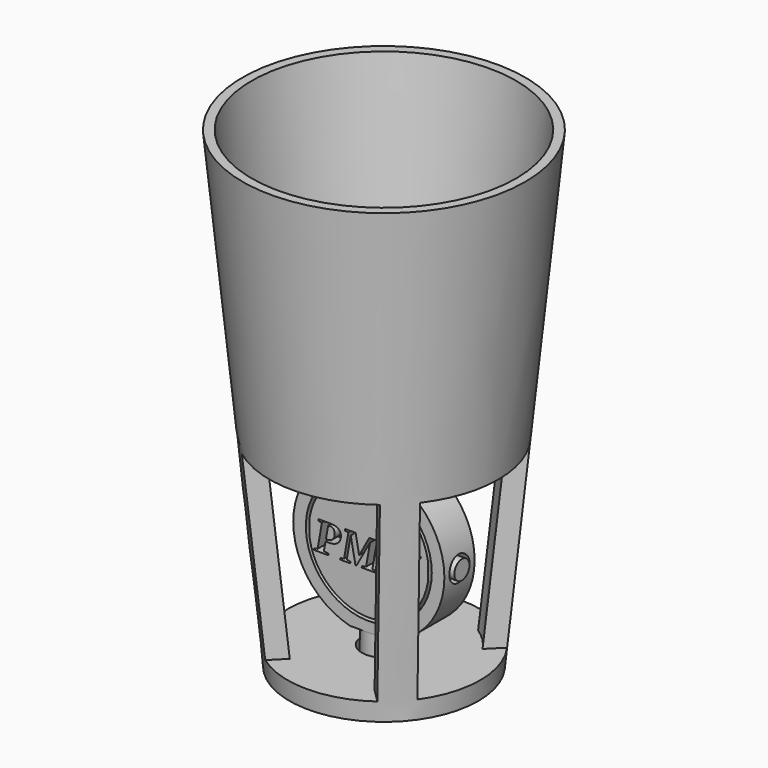
from build123d import *

# Parameters (mm, degrees)
F3_DEPTH      = 29
F4_R          = 3.5
F5_DEPTH      = 2
F5_DEPTH_BACK = 31
F6_R          = 10
F7_DEPTH      = 3
F8_R          = 2
F9_DEPTH      = 15
F11_DEPTH     = 3
F16_TEXT_SIZE = 6.9444444444
F17_DEPTH     = 2
F18_TEXT_SIZE = 6.9444444444
F19_DEPTH     = 2


# Not quite as in the source:
# - Text() gives the source's letters only with a copy of the font that has no kerning and outlines rounded to 1/6400 em; it was checked with that copy


with BuildPart() as f1:
    # F0 (on Front) → F1 (revolve)
    with BuildSketch(Plane.XZ):
        Polygon((0, 3), (0, 0), (15, 0), (22.447081343, 75), (21, 75), (17.0282232837, 35), (0, 35), (0, 32), (15.1626685751, 32), (12.2831304558, 3), align=None)
    revolve(axis=Axis((0, 0, 33.5), (0, 0, 1)))

    # F2 (on face) → F3 (cut)
    with BuildSketch(Plane.XY.offset(3)):
        with BuildLine():
            Line((12.2634482474, 15.7989821534), (15.6845353346, 19.2200692405))
            ThreePointArc((15.6845353346, 19.2200692405), (0, 24.8075736474), (-15.6845353346, 19.2200692405))
            Line((-15.6845353346, 19.2200692405), (-12.2634482474, 15.7989821534))
            Line((-12.2634482474, 15.7989821534), (-5.0787650158, 8.6142989218))
            ThreePointArc((-5.0787650158, 8.6142989218), (0, 10), (5.0787650158, 8.6142989218))
            Line((5.0787650158, 8.6142989218), (12.2634482474, 15.7989821534))
        make_face()
        with BuildLine():
            Line((19.2200692405, 15.6845353346), (15.7989821534, 12.2634482474))
            Line((15.7989821534, 12.2634482474), (8.6142989218, 5.0787650158))
            ThreePointArc((8.6142989218, 5.0787650158), (10, 0), (8.6142989218, -5.0787650158))
            Line((8.6142989218, -5.0787650158), (15.7989821534, -12.2634482474))
            Line((15.7989821534, -12.2634482474), (19.2200692405, -15.6845353346))
            ThreePointArc((19.2200692405, -15.6845353346), (24.8075736474, 0), (19.2200692405, 15.6845353346))
        make_face()
        with BuildLine():
            Line((-8.6142989218, 5.0787650158), (-15.7989821534, 12.2634482474))
            Line((-15.7989821534, 12.2634482474), (-19.2200692405, 15.6845353346))
            ThreePointArc((-19.2200692405, 15.6845353346), (-24.8075736474, 0), (-19.2200692405, -15.6845353346))
            Line((-19.2200692405, -15.6845353346), (-15.7989821534, -12.2634482474))
            Line((-15.7989821534, -12.2634482474), (-8.6142989218, -5.0787650158))
            ThreePointArc((-8.6142989218, -5.0787650158), (-10, 0), (-8.6142989218, 5.0787650158))
        make_face()
        with BuildLine():
            Line((15.6845353346, -19.2200692405), (12.2634482474, -15.7989821534))
            Line((12.2634482474, -15.7989821534), (5.0787650158, -8.6142989218))
            ThreePointArc((5.0787650158, -8.6142989218), (0, -10), (-5.0787650158, -8.6142989218))
            Line((-5.0787650158, -8.6142989218), (-12.2634482474, -15.7989821534))
            Line((-12.2634482474, -15.7989821534), (-15.6845353346, -19.2200692405))
            ThreePointArc((-15.6845353346, -19.2200692405), (0, -24.8075736474), (15.6845353346, -19.2200692405))
        make_face()
    extrude(amount=F3_DEPTH, mode=Mode.SUBTRACT)

    # F4 (on face) → F5 (cut, two sides)
    with BuildSketch(Plane.XY.offset(3)) as f5_sk:
        Circle(F4_R)
    extrude(amount=-F5_DEPTH, mode=Mode.SUBTRACT)
    extrude(f5_sk.sketch, amount=F5_DEPTH_BACK, mode=Mode.SUBTRACT)


with BuildPart() as f7:
    # F6 (on Front) → F7 (new body, symmetric)
    with BuildSketch(Plane.XZ):
        with BuildLine():
            Line((3, 33.25), (0, 33.25))
            Line((0, 33.25), (-3, 33.25))
            Line((-3, 33.25), (-3, 29.1189500386))
            ThreePointArc((-3, 29.1189500386), (-12, 17.5), (-3, 5.8810499614))
            Line((-3, 5.8810499614), (-3, 1.75))
            Line((-3, 1.75), (0, 1.75))
            Line((0, 1.75), (3, 1.75))
            Line((3, 1.75), (3, 5.8810499614))
            ThreePointArc((3, 5.8810499614), (12, 17.5), (3, 29.1189500386))
            Line((3, 29.1189500386), (3, 33.25))
        make_face()
        with Locations((0, 17.5)):
            Circle(F6_R, mode=Mode.SUBTRACT)
    extrude(amount=F7_DEPTH, both=True)

    # F8 (on Right) → F9 (cut, symmetric)
    with BuildSketch(Plane.YZ):
        with Locations((0, 17.5)):
            Circle(F8_R)
    extrude(amount=F9_DEPTH, both=True, mode=Mode.SUBTRACT)

    # F12 (on Front) → F13 (revolve, cut)
    with BuildSketch(Plane.XZ):
        Polygon((0, 33.25), (3, 33.25), (3, 29.1189500386), (5, 29.1189500386), (5, 34.3002825975), (0, 34.3002825975), align=None)
        Polygon((5, 0.6997174025), (5, 5.8810499614), (3, 5.8810499614), (3, 1.75), (0, 1.75), (0, 0.6997174025), align=None)
    revolve(axis=Axis((0, 0, 33.7751412988), (0, 0, 1)), mode=Mode.SUBTRACT)


with BuildPart() as f11:
    # F10 (on Front) → F11 (new body, symmetric)
    with BuildSketch(Plane.XZ):
        with BuildLine():
            Line((12.3808315196, 19), (9.3808315196, 19))
            ThreePointArc((9.3808315196, 19), (0, 27), (-9.3808315196, 19))
            Line((-9.3808315196, 19), (-12.3808315196, 19))
            Line((-12.3808315196, 19), (-12.3808315196, 17.5))
            Line((-12.3808315196, 17.5), (-12.3808315196, 16))
            Line((-12.3808315196, 16), (-9.3808315196, 16))
            ThreePointArc((-9.3808315196, 16), (0, 8), (9.3808315196, 16))
            Line((9.3808315196, 16), (12.3808315196, 16))
            Line((12.3808315196, 16), (12.3808315196, 17.5))
            Line((12.3808315196, 17.5), (12.3808315196, 19))
        make_face()
    extrude(amount=F11_DEPTH, both=True)

    # F14 (on Front) → F15 (revolve, cut)
    with BuildSketch(Plane.XZ):
        Polygon((9.3808315196, 22.3522800952), (9.3808315196, 19), (12.3808315196, 19), (12.3808315196, 17.5), (14.9963386357, 17.5), (14.9963386357, 22.3522800952), align=None)
        Polygon((-14.9963386357, 17.5), (-12.3808315196, 17.5), (-12.3808315196, 19), (-9.3808315196, 19), (-9.3808315196, 22.3522800952), (-14.9963386357, 22.3522800952), align=None)
    revolve(axis=Axis((-13.6885850777, 0, 17.5), (1, 0, 0)), mode=Mode.SUBTRACT)

    # F16 (on face) → F17 (cut)
    with BuildSketch(Plane.XZ.offset(3)):
        with Locations((-8.7179904514, 14.6233281703)):
            Text('PMW', F16_TEXT_SIZE, font='Tinos', font_style=FontStyle.BOLDITALIC, text_align=(TextAlign.LEFT, TextAlign.BOTTOM))
    extrude(amount=-F17_DEPTH, mode=Mode.SUBTRACT)

    # F18 (on face) → F19 (cut)
    with BuildSketch(Plane(origin=(0, 3, 0), x_dir=(-1, 0, 0), z_dir=(0, 1, 0))):
        with Locations((-3.8471137153, 20.4582289754)):
            Text('21', F18_TEXT_SIZE, font='Tinos', font_style=FontStyle.BOLDITALIC, text_align=(TextAlign.LEFT, TextAlign.BOTTOM))
        with Locations((-7.3193359375, 12.4721178643)):
            Text('2017', F18_TEXT_SIZE, font='Tinos', font_style=FontStyle.BOLDITALIC, text_align=(TextAlign.LEFT, TextAlign.BOTTOM))
    extrude(amount=-F19_DEPTH, mode=Mode.SUBTRACT)


with BuildPart() as f21:
    # F20 (on Front) → F21 (revolve)
    with BuildSketch(Plane.XZ):
        Polygon((20.4986119055, 69.9504906211), (20.9975468235, 74.9752939134), (0, 74.9752939134), (0, 34.9752939134), (17.0257701072, 34.9752939134), align=None)
    revolve(axis=Axis((0, 0, 54.9752939134), (0, 0, -1)))


solid = Compound([f1.part, f7.part, f11.part])
